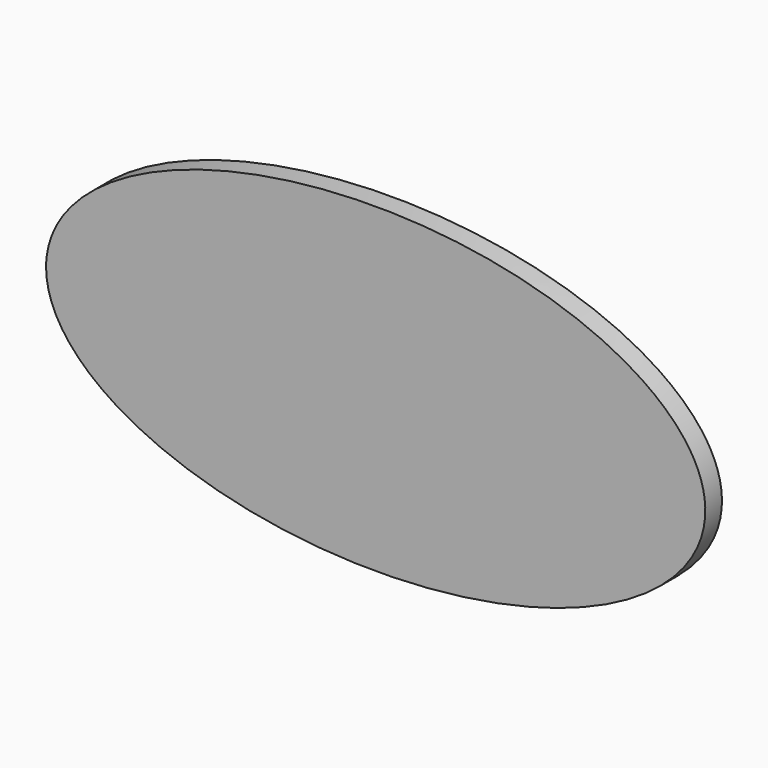
from build123d import *

# Parameters (mm, degrees)
F1_DEPTH = 2.0066


# Not quite as in the source:
# - the program builds the solid bodies; features that only make, move or delete a surface that nothing else refers to are left out


with BuildPart() as f1:
    # F0 (on Front) → F1 (new body)
    with BuildSketch(Plane.XZ):
        with BuildLine():
            add(Edge.make_bspline(
                [(-31.75, 0), (-31.75, -26.7865598037), (15.875, -13.3932799019), (63.5, 0), (15.875, 13.3932799019), (-31.75, 26.7865598037), (-31.75, 0)],
                knots=[0, 0, 0, 2.0943951024, 2.0943951024, 4.1887902048, 4.1887902048, 6.2831853072, 6.2831853072, 6.2831853072], degree=2, weights=[1, 0.5, 1, 0.5, 1, 0.5, 1]))
        make_face()
    extrude(amount=F1_DEPTH)


solid = f1.part
